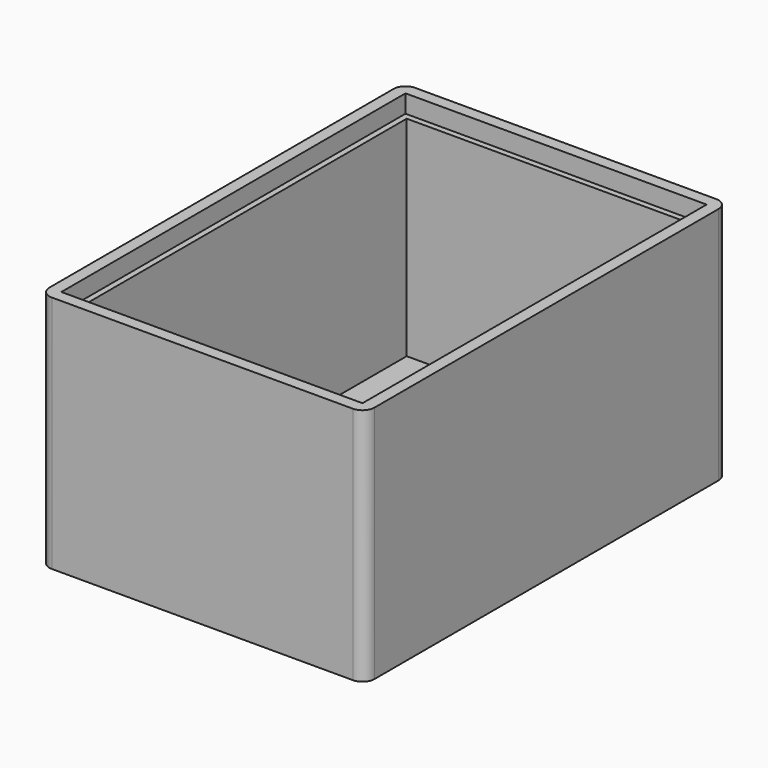
from build123d import *

# Parameters (mm, degrees)
F1_DEPTH = 127
F2_T     = 6.35
F3_W     = 160.02
F3_H     = 228.6
F3_W_2   = 153.67
F3_H_2   = 222.25
F4_DEPTH = 127
F5_DEPTH = 9.525
F6_R     = 1.5875
F7_DEPTH = 25.4
F8_W     = 29.6064093709
F8_H     = 23.796312511
F9_DEPTH = 25.4


# Not quite as in the source:
# - a shell that OpenCascade refuses in one call is made with other operations: the cavity is built on its own and cut out


with BuildPart() as f1:
    # F0 (on Top) → F1 (new body)
    with BuildSketch(Plane.XY):
        with BuildLine():
            ThreePointArc((-33.8929891586, 6.35), (-32.0331172192, 1.8598719395), (-27.5429891586, 0))
            Line((-27.5429891586, 0), (132.4770108414, 0))
            ThreePointArc((132.4770108414, 0), (136.9671389019, 1.8598719395), (138.8270108414, 6.35))
            Line((138.8270108414, 6.35), (138.8270108414, 234.95))
            ThreePointArc((138.8270108414, 234.95), (136.9671389019, 239.4401280605), (132.4770108414, 241.3))
            Line((132.4770108414, 241.3), (-27.5429891586, 241.3))
            ThreePointArc((-27.5429891586, 241.3), (-32.0331172192, 239.4401280605), (-33.8929891586, 234.95))
            Line((-33.8929891586, 234.95), (-33.8929891586, 6.35))
        make_face()
    extrude(amount=F1_DEPTH)

    # F2: shell of thickness 6.35, made by hand


with BuildPart() as f2_core1:
    # F2_t2: copy of F1
    add(f1.part)

    # the walls: a layer under each face that stays
    f2_faces = [f2_core1.faces().sort_by_distance(p)[0] for p in [
        (52.4670108414, 0, 63.5),
        (138.8270108414, 120.65, 63.5),
        (52.4670108414, 241.3, 63.5),
        (-33.8929891586, 120.65, 63.5),
        (52.4670108414, 120.65, 0),
    ]]
    thicken(f2_faces, amount=-F2_T, mode=Mode.SUBTRACT)


with BuildPart() as f1_1:
    add(f1.part)

    # what is left inside the walls is the cavity
    f2_cavity = [f2_core1.part.solids().sort_by_distance(p)[0] for p in [
        (52.467011, 82.55, 6.4135),
    ]]
    add(f2_cavity, mode=Mode.SUBTRACT)

    # F3 (on face) → F4 (join)
    with BuildSketch(Plane.XY.offset(127)):
        with Locations((52.4670108414, 120.65)):
            Rectangle(F3_W, F3_H)
        with Locations((52.4670108414, 120.65)):
            Rectangle(F3_W_2, F3_H_2, mode=Mode.SUBTRACT)
    extrude(amount=-F4_DEPTH)

    # F3 (on face) → F5 (cut)
    with BuildSketch(Plane.XY.offset(127)):
        with Locations((52.4670108414, 120.65)):
            Rectangle(F3_W, F3_H)
        with Locations((52.4670108414, 120.65)):
            Rectangle(F3_W_2, F3_H_2, mode=Mode.SUBTRACT)
    extrude(amount=-F5_DEPTH, mode=Mode.SUBTRACT)

    # F6 (on face) → F7 (cut)
    with BuildSketch(Plane(origin=(0, 0, 0), x_dir=(1, 0, 0), z_dir=(0, 0, -1))):
        with Locations((-0.9629237612, -29.5858253049)):
            Circle(F6_R)
    extrude(amount=-F7_DEPTH, mode=Mode.SUBTRACT)

    # F8 (on face) → F9 (cut)
    with BuildSketch(Plane(origin=(0, 0, 0), x_dir=(1, 0, 0), z_dir=(0, 0, -1))):
        with Locations((25.6846360862, -31.3592217863)):
            Rectangle(F8_W, F8_H)
    extrude(amount=-F9_DEPTH, mode=Mode.SUBTRACT)


solid = f1_1.part
